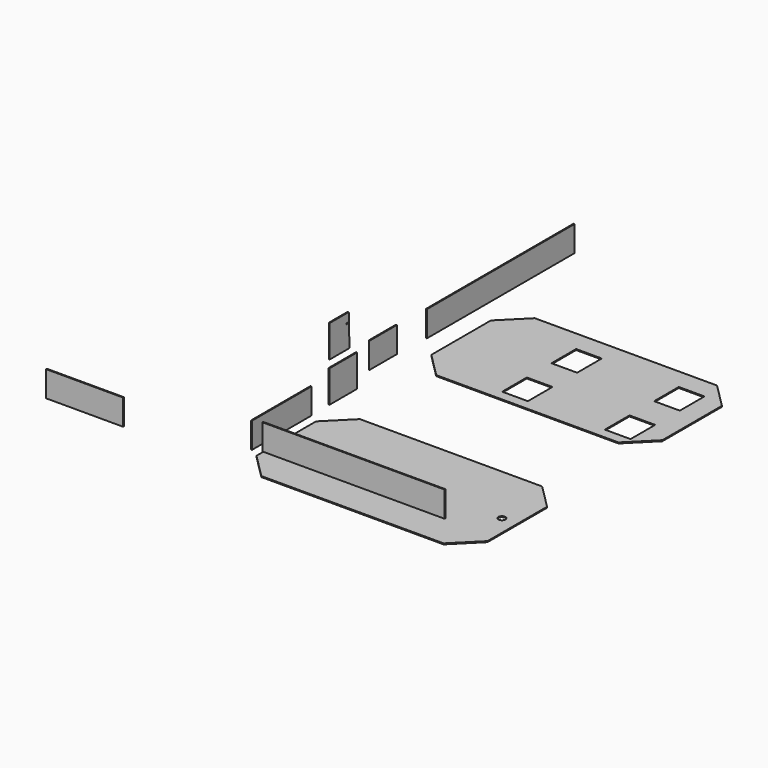
from build123d import *

# Parameters (mm, degrees)
F0_W      = 2438.4
F0_H      = 1219.2
F1_DEPTH  = 9.525
F3_DEPTH  = 25.4
F5_DEPTH  = 25.4
F6_W      = 736.6
F6_H      = 254
F7_DEPTH  = 9.525
F8_W      = 1803.4
F8_H      = 254
F9_DEPTH  = 9.525
F10_W     = 736.6
F10_H     = 317.5
F11_DEPTH = 9.525
F12_W     = 254
F12_H     = 317.5
F13_DEPTH = 9.525
F15_DEPTH = 317.5
F18_DEPTH = 330.2
F19_R     = 6.35
F20_DEPTH = 25.4
F21_W     = 342.9
F21_H     = 317.5
F23_DEPTH = 9.525
F22_W     = 342.9
F22_H     = 254
F24_DEPTH = 9.525
F25_W     = 2286
F25_H     = 1219.2
F26_DEPTH = 9.525
F28_DEPTH = 25.4
F30_W     = 33.3816595376
F30_H     = 808.2542568445
F31_DEPTH = 25.4
F32_W     = 1828.8
F32_H     = 254
F33_DEPTH = 9.525
F34_W     = 762
F34_H     = 254
F35_DEPTH = 9.525
F37_DEPTH = 254
F38_W     = 254
F38_H     = 304.8
F39_DEPTH = 101.6
F40_R     = 34.925
F41_DEPTH = 127


# Not quite as in the source:
# - a feature names something its author has since deleted; it is built from what else it names


with BuildPart() as f1:
    # F0 (on Top) → F1 (new body)
    with BuildSketch(Plane.XY):
        with Locations((1219.2, 609.6)):
            Rectangle(F0_W, F0_H)
    extrude(amount=F1_DEPTH)

    # F2 (on face) → F3 (cut)
    with BuildSketch(Plane.XY.offset(9.525)):
        Polygon((0, 1219.2), (0, 977.9), (241.3, 1219.2), align=None)
        Polygon((241.3, 0), (0, 241.3), (0, 0), align=None)
    extrude(amount=-F3_DEPTH, mode=Mode.SUBTRACT)

    # F4 (on face) → F5 (cut)
    with BuildSketch(Plane.XY.offset(9.525)):
        Polygon((2438.4, 0), (2438.4, 1219.2), (2044.7, 1219.2), (2285.9994819731, 977.9005180269), (2285.9994819731, 241.2994819731), (2044.7, 0), align=None)
    extrude(amount=-F5_DEPTH, mode=Mode.SUBTRACT)

    # F30 (on face) → F31 (cut)
    with BuildSketch(Plane(origin=(-0.1994328009, 0, 9.5208224783), x_dir=(0.9997806835, 0, 0.0209424199), z_dir=(-0.0209424199, 0, 0.9997806835))):
        with Locations((-16.6908297688, 615.603916347)):
            Rectangle(F30_W, F30_H)
    extrude(amount=-F31_DEPTH, mode=Mode.SUBTRACT)

    # F40 (on face) → F41 (cut)
    with BuildSketch(Plane(origin=(-0.1994328009, 0, 9.5208224783), x_dir=(0.9997806835, 0, 0.0209424199), z_dir=(-0.0209424199, 0, 0.9997806835))):
        with Locations((2133.2976010596, 609.6)):
            Circle(F40_R)
    extrude(amount=-F41_DEPTH, mode=Mode.SUBTRACT)


with BuildPart() as f7:
    # F6 (on Right) → F7 (new body)
    with BuildSketch(Plane.YZ):
        with Locations((540.855868909, 217.8485281765)):
            Rectangle(F6_W, F6_H)
    extrude(amount=F7_DEPTH)


with BuildPart() as f9:
    # F8 (on Front) → F9 (new body)
    with BuildSketch(Plane.XZ):
        with Locations((1152.5721657038, 353.8724693788)):
            Rectangle(F8_W, F8_H)
    extrude(amount=-F9_DEPTH)


with BuildPart() as f11:
    # F10 (on Right) → F11 (new body)
    with BuildSketch(Plane.YZ):
        with Locations((396.9467690647, 657.1327268381)):
            Rectangle(F10_W, F10_H)
    extrude(amount=F11_DEPTH)


with BuildPart() as f13:
    # F12 (on Right) → F13 (new body)
    with BuildSketch(Plane.YZ):
        with Locations((1257.1182154525, 646.2227201939)):
            Rectangle(F12_W, F12_H)
    extrude(amount=F13_DEPTH)

    # F14 (on face) → F15 (cut)
    with BuildSketch(Plane.XY.offset(804.9727201939)):
        Polygon((0, 1130.1182154525), (9.525, 1130.1182154525), (0, 1139.6432154525), align=None)
    extrude(amount=-F15_DEPTH, mode=Mode.SUBTRACT)

    # F17 (on face) → F18 (cut)
    with BuildSketch(Plane(origin=(0, -13.2369765094, 446.0001862794), x_dir=(1, 0, 0), z_dir=(0, 0.0296662441, -0.9995598601))):
        Polygon((10.085565038, -1394.4936855086), (9.5443632454, -1393.981218338), (0, -1384.9436044693), (0, -1420.4403162003), (10.085565038, -1420.4403162003), align=None)
    extrude(amount=-F18_DEPTH, mode=Mode.SUBTRACT)

    # F19 (on face) → F20 (cut)
    with BuildSketch(Plane.YZ.offset(9.525)):
        with Locations((1349.4267463684, 713.9506340027)):
            Circle(F19_R)
    extrude(amount=-F20_DEPTH, mode=Mode.SUBTRACT)


with BuildPart() as f23:
    # F21 (on Right) → F23 (new body)
    with BuildSketch(Plane.YZ):
        with Locations((1302.5214076042, 252.6165406551)):
            Rectangle(F21_W, F21_H)
    extrude(amount=F23_DEPTH)


with BuildPart() as f24:
    # F22 (on Right) → F24 (new body)
    with BuildSketch(Plane.YZ):
        with Locations((1795.0915694237, 323.2190309106)):
            Rectangle(F22_W, F22_H)
    extrude(amount=F24_DEPTH)

    # F36 (on face) → F37 (cut)
    with BuildSketch(Plane.XY.offset(450.2190309106)):
        Polygon((0, 1957.0165694237), (9.525, 1966.5415694237), (0, 1966.5415694237), align=None)
        Polygon((0, 1623.6415694237), (9.525, 1623.6415694237), (0, 1633.1665694237), align=None)
    extrude(amount=-F37_DEPTH, mode=Mode.SUBTRACT)


with BuildPart() as f26:
    # F25 (on Top) → F26 (new body)
    with BuildSketch(Plane.XY):
        with Locations((1143, 2772.41582157)):
            Rectangle(F25_W, F25_H)
    extrude(amount=F26_DEPTH)

    # F27 (on face) → F28 (cut)
    with BuildSketch(Plane.XY.offset(9.525)):
        Polygon((241.3, 3382.01582157), (0, 3382.01582157), (0, 3140.71582157), align=None)
        Polygon((241.3, 2162.81582157), (0, 2404.11582157), (0, 2162.81582157), align=None)
        Polygon((2286, 3382.01582157), (2044.7, 3382.01582157), (2286, 3140.71582157), align=None)
        Polygon((2286, 2162.81582157), (2286, 2404.11582157), (2044.7, 2162.81582157), align=None)
    extrude(amount=-F28_DEPTH, mode=Mode.SUBTRACT)

    # F38 (on face) → F39 (cut)
    with BuildSketch(Plane.XY.offset(9.525)):
        with Locations((939.8, 3026.41582157)):
            Rectangle(F38_W, F38_H)
        with Locations((939.8, 2416.81582157)):
            Rectangle(F38_W, F38_H)
        with Locations((1955.8, 3026.41582157)):
            Rectangle(F38_W, F38_H)
        with Locations((1955.8, 2416.81582157)):
            Rectangle(F38_W, F38_H)
    extrude(amount=-F39_DEPTH, mode=Mode.SUBTRACT)


with BuildPart() as f33:
    # F32 (on Right) → F33 (new body)
    with BuildSketch(Plane.YZ):
        with Locations((3251.0826839447, 309.7931716245)):
            Rectangle(F32_W, F32_H)
    extrude(amount=F33_DEPTH)


with BuildPart() as f35:
    # F34 (on Front) → F35 (new body)
    with BuildSketch(Plane.XZ):
        with Locations((-1499.9832916029, 127)):
            Rectangle(F34_W, F34_H)
    extrude(amount=F35_DEPTH)


solid = Compound([f1.part, f7.part, f9.part, f13.part, f23.part, f24.part, f26.part, f33.part, f35.part])
